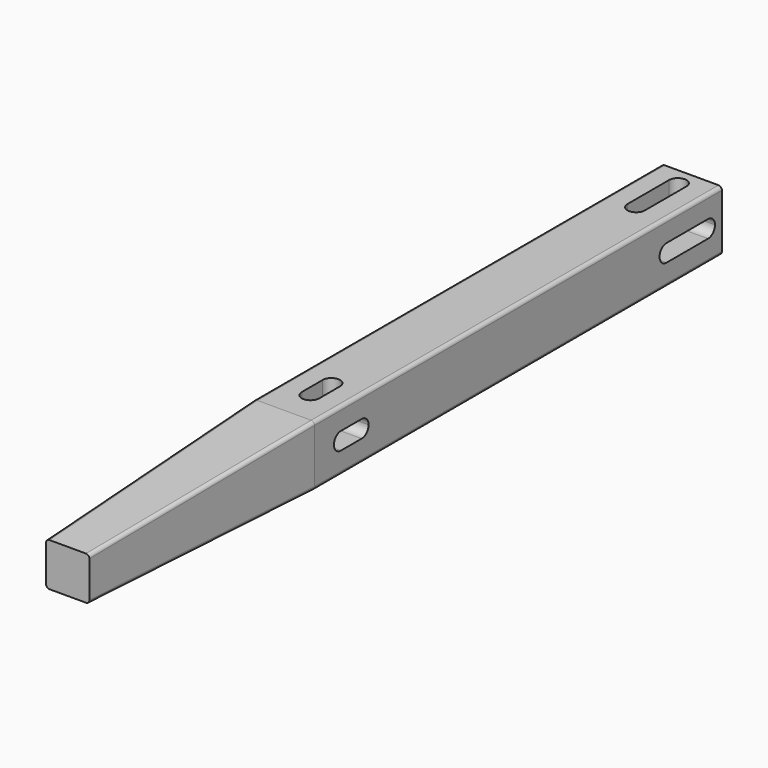
from build123d import *

# Parameters (mm, degrees)
F0_W         = 35
F0_H         = 35
F1_DEPTH     = 444
F3_DEPTH     = 35
F5_DEPTH     = 35
F7_DEPTH     = 17.5
F10_DEPTH    = 17.5
F11_T1_DEPTH = 160.3329637837
F11_T3_DEPTH = 304
F11_T5_DEPTH = 160.3329637837
F11_T7_DEPTH = 160.6210414072
F11_T9_DEPTH = 454


# Not quite as in the source:
# - a fillet or chamfer that OpenCascade refuses, or shapes differently, is made with other operations: its cross-section is extruded or revolved along the edge and cut away or added


with BuildPart() as f1:
    # F0 (on Front) → F1 (new body)
    with BuildSketch(Plane.XZ):
        Rectangle(F0_W, F0_H)
    extrude(amount=F1_DEPTH)

    # F2 (on face) → F3 (cut)
    with BuildSketch(Plane.YZ.offset(17.5)):
        Polygon((-444, 7.5), (-294, 17.5), (-444, 17.5), align=None)
    extrude(amount=-F3_DEPTH, mode=Mode.SUBTRACT)

    # F4 (on face) → F5 (cut)
    with BuildSketch(Plane.XY.offset(17.5)):
        Polygon((17.5, -444), (17.5, -294), (7.5, -444), align=None)
    extrude(amount=-F5_DEPTH, mode=Mode.SUBTRACT)

    # F6 (on face) → F7 (cut)
    with BuildSketch(Plane.XY.offset(17.5)):
        with BuildLine():
            ThreePointArc((5, -275), (0, -270), (-5, -275))
            Line((-5, -275), (5, -275))
        make_face()
        with BuildLine():
            Line((-5, -260), (-5, -275))
            ThreePointArc((-5, -275), (0, -270), (5, -275))
            Line((5, -275), (5, -260))
            ThreePointArc((5, -260), (0, -265), (-5, -260))
        make_face()
        with BuildLine():
            Line((5, -275), (-5, -275))
            ThreePointArc((-5, -275), (0, -280), (5, -275))
        make_face()
        with BuildLine():
            ThreePointArc((5, -260), (0, -255), (-5, -260))
            Line((-5, -260), (5, -260))
        make_face()
        with BuildLine():
            Line((5, -260), (-5, -260))
            ThreePointArc((-5, -260), (0, -265), (5, -260))
        make_face()
        with BuildLine():
            ThreePointArc((5, -40), (0, -35), (-5, -40))
            Line((-5, -40), (5, -40))
        make_face()
        with BuildLine():
            Line((-5, -10), (-5, -40))
            ThreePointArc((-5, -40), (0, -35), (5, -40))
            Line((5, -40), (5, -10))
            ThreePointArc((5, -10), (0, -15), (-5, -10))
        make_face()
        with BuildLine():
            Line((5, -40), (-5, -40))
            ThreePointArc((-5, -40), (0, -45), (5, -40))
        make_face()
        with BuildLine():
            ThreePointArc((5, -10), (0, -5), (-5, -10))
            Line((-5, -10), (5, -10))
        make_face()
        with BuildLine():
            Line((5, -10), (-5, -10))
            ThreePointArc((-5, -10), (0, -15), (5, -10))
        make_face()
    extrude(amount=-F7_DEPTH, mode=Mode.SUBTRACT)

    # F9 (on face) → F10 (cut)
    with BuildSketch(Plane.YZ.offset(17.5)):
        with BuildLine():
            ThreePointArc((-270, 0), (-271.4644660941, -3.5355339059), (-275, -5))
            Line((-275, -5), (-260, -5))
            ThreePointArc((-260, -5), (-265, 0), (-260, 5))
            Line((-260, 5), (-275, 5))
            ThreePointArc((-275, 5), (-271.4644660941, 3.5355339059), (-270, 0))
        make_face()
        with BuildLine():
            ThreePointArc((-275, 5), (-280, 0), (-275, -5))
            Line((-275, -5), (-275, 5))
        make_face()
        with BuildLine():
            Line((-275, 5), (-275, -5))
            ThreePointArc((-275, -5), (-271.4644660941, -3.5355339059), (-270, 0))
            ThreePointArc((-270, 0), (-271.4644660941, 3.5355339059), (-275, 5))
        make_face()
        with BuildLine():
            ThreePointArc((-260, 5), (-265, 0), (-260, -5))
            Line((-260, -5), (-260, 5))
        make_face()
        with BuildLine():
            Line((-260, 5), (-260, -5))
            ThreePointArc((-260, -5), (-256.4644660941, -3.5355339059), (-255, 0))
            ThreePointArc((-255, 0), (-256.4644660941, 3.5355339059), (-260, 5))
        make_face()
        with BuildLine():
            ThreePointArc((-35, 0), (-36.4644660941, -3.5355339059), (-40, -5))
            Line((-40, -5), (-10, -5))
            ThreePointArc((-10, -5), (-15, 0), (-10, 5))
            Line((-10, 5), (-40, 5))
            ThreePointArc((-40, 5), (-36.4644660941, 3.5355339059), (-35, 0))
        make_face()
        with BuildLine():
            ThreePointArc((-40, 5), (-45, 0), (-40, -5))
            Line((-40, -5), (-40, 5))
        make_face()
        with BuildLine():
            Line((-40, 5), (-40, -5))
            ThreePointArc((-40, -5), (-36.4644660941, -3.5355339059), (-35, 0))
            ThreePointArc((-35, 0), (-36.4644660941, 3.5355339059), (-40, 5))
        make_face()
        with BuildLine():
            ThreePointArc((-10, 5), (-15, 0), (-10, -5))
            Line((-10, -5), (-10, 5))
        make_face()
        with BuildLine():
            Line((-10, 5), (-10, -5))
            ThreePointArc((-10, -5), (-6.4644660941, -3.5355339059), (-5, 0))
            ThreePointArc((-5, 0), (-6.4644660941, 3.5355339059), (-10, 5))
        make_face()
    extrude(amount=-F10_DEPTH, mode=Mode.SUBTRACT)

    # F11: fillet of radius 2 on 7 edges, made by hand

    # F11_s2 → F11_t1 (cut)
    with BuildSketch(Plane(origin=(0, -446.5265364088, -29.7684357606), x_dir=(1, 0, 0), z_dir=(0, 0.9977851579, 0.0665190105))):
        with BuildLine():
            ThreePointArc((-17.5, -35.0178293565), (-16.9142135624, -36.4320429189), (-15.5, -37.0178293565))
            Line((-15.5, -37.0178293565), (-17.5, -37.0178293565))
            Line((-17.5, -37.0178293565), (-17.5, -35.0178293565))
        make_face()
    extrude(amount=F11_T1_DEPTH, mode=Mode.SUBTRACT)

    # F11_s4 → F11_t3 (cut)
    with BuildSketch(Plane.XZ.offset(-5)):
        with BuildLine():
            ThreePointArc((-17.5, 15.5), (-16.9142135624, 16.9142135624), (-15.5, 17.5))
            Line((-15.5, 17.5), (-17.5, 17.5))
            Line((-17.5, 17.5), (-17.5, 15.5))
        make_face()
        with BuildLine():
            ThreePointArc((15.5, 17.5), (16.9142135624, 16.9142135624), (17.5, 15.5))
            Line((17.5, 15.5), (17.5, 17.5))
            Line((17.5, 17.5), (15.5, 17.5))
        make_face()
        with BuildLine():
            ThreePointArc((15.5, -17.5), (16.9142135624, -16.9142135624), (17.5, -15.5))
            Line((17.5, -15.5), (17.5, -17.5))
            Line((17.5, -17.5), (15.5, -17.5))
        make_face()
    extrude(amount=F11_T3_DEPTH, mode=Mode.SUBTRACT)

    # F11_s6 → F11_t5 (cut)
    with BuildSketch(Plane(origin=(-19.1032456553, -286.5486848302, 0), x_dir=(0, 0, 1), z_dir=(-0.0665190105, -0.9977851579, 0))):
        with BuildLine():
            ThreePointArc((-17.5, -35.0178293565), (-16.9142135624, -36.4320429189), (-15.5, -37.0178293565))
            Line((-15.5, -37.0178293565), (-17.5, -37.0178293565))
            Line((-17.5, -37.0178293565), (-17.5, -35.0178293565))
        make_face()
    extrude(amount=F11_T5_DEPTH, mode=Mode.SUBTRACT)

    # F11_s8 → F11_t7 (cut)
    with BuildSketch(Plane(origin=(-29.6035242291, -444.0528634361, -29.6035242291), x_dir=(-0.9977851579, 0.0665190105, 0), z_dir=(0.0663723312, 0.9955849674, 0.0663723312))):
        with BuildLine():
            ThreePointArc((-35.026678914, 36.8632049195), (-36.4351682565, 36.2743058009), (-37.0178293565, 34.8632244983))
            Line((-37.0178293565, 34.8632244983), (-37.0178293565, 36.8543944331))
            Line((-37.0178293565, 36.8543944331), (-35.026678914, 36.8632049195))
        make_face()
    extrude(amount=F11_T7_DEPTH, mode=Mode.SUBTRACT)

    # F11_s10 → F11_t9 (cut)
    with BuildSketch(Plane.XZ.offset(-5)):
        with BuildLine():
            ThreePointArc((-17.5, -15.5), (-16.9142135624, -16.9142135624), (-15.5, -17.5))
            Line((-15.5, -17.5), (-17.5, -17.5))
            Line((-17.5, -17.5), (-17.5, -15.5))
        make_face()
    extrude(amount=F11_T9_DEPTH, mode=Mode.SUBTRACT)


solid = f1.part
